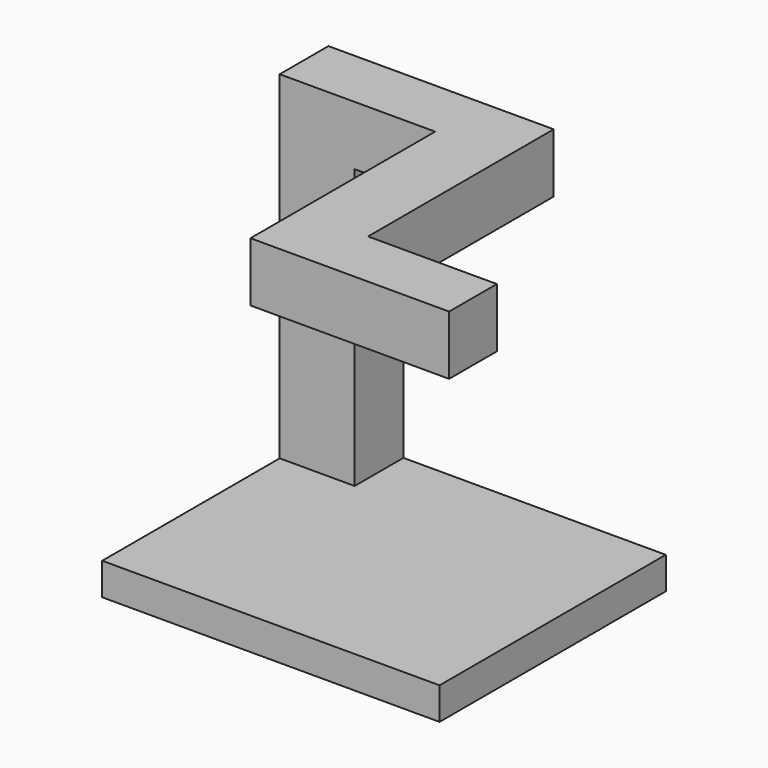
from build123d import *

# Parameters (mm, degrees)
F0_W     = 62.8466829658
F0_H     = 52.6766888797
F1_DEPTH = 6
F2_W     = 13.9663396403
F2_H     = 11.3499658182
F3_DEPTH = 63
F4_W     = 11.3499658182
F4_H     = 11.0394264162
F5_DEPTH = 28
F6_W     = 13.0074043497
F6_H     = 11.0394264162
F7_DEPTH = 43
F8_W     = 11.1150065735
F8_H     = 11.0394264162
F9_DEPTH = 24


with BuildPart() as f1:
    # F0 (on Top) → F1 (new body)
    with BuildSketch(Plane.XY):
        with Locations((2.4644061923, -3.5718083382)):
            Rectangle(F0_W, F0_H)
    extrude(amount=F1_DEPTH)

    # F2 (on face) → F3 (join)
    with BuildSketch(Plane.XY.offset(6)):
        with Locations((-21.9757654704, 17.0915531926)):
            Rectangle(F2_W, F2_H)
    extrude(amount=F3_DEPTH)

    # F4 (on face) → F5 (join)
    with BuildSketch(Plane.YZ.offset(-14.9925956503)):
        with Locations((17.0915531926, 63.4802867919)):
            Rectangle(F4_W, F4_H)
    extrude(amount=F5_DEPTH)

    # F6 (on face) → F7 (join)
    with BuildSketch(Plane.XZ.offset(-11.4165702835)):
        with Locations((6.5037021749, 63.4802867919)):
            Rectangle(F6_W, F6_H)
    extrude(amount=F7_DEPTH)

    # F8 (on face) → F9 (join)
    with BuildSketch(Plane.YZ.offset(13.0074043497)):
        with Locations((-26.0259264298, 63.4802867919)):
            Rectangle(F8_W, F8_H)
    extrude(amount=F9_DEPTH)


solid = f1.part
